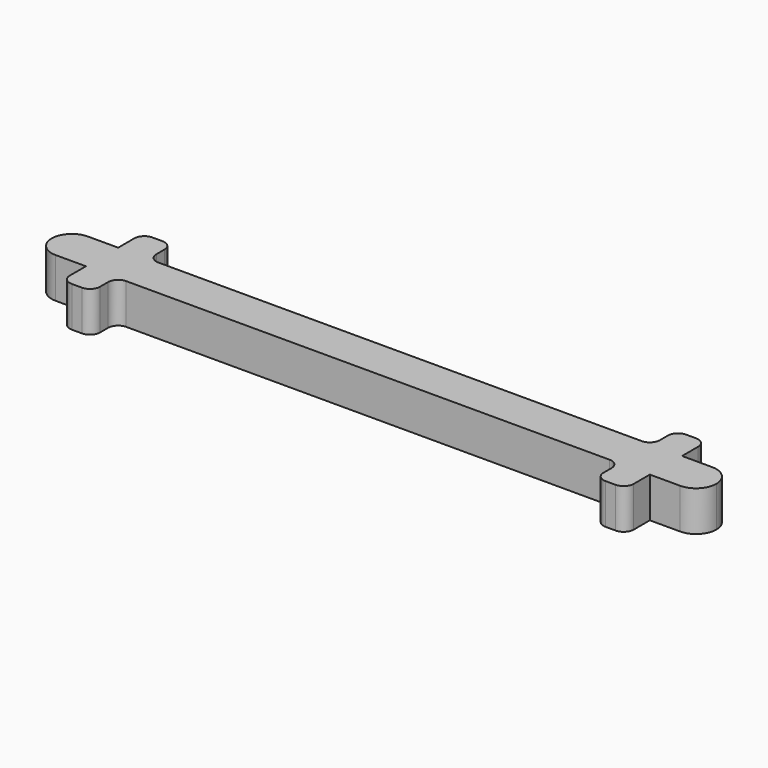
from build123d import *

# Parameters (mm, degrees)
F1_DEPTH = 4
F2_R     = 1.99999
F3_R     = 1


# Not quite as in the source:
# - a fillet or chamfer is up to 0.001 mm smaller than in the source, because OpenCascade refuses the exact size


with BuildPart() as f1:
    # F0 (on Top) → F1 (new body)
    with BuildSketch(Plane.XY):
        Polygon((-28, 2), (-33, 2), (-33, -2), (-28, -2), (-28, -5), (-25, -5), (-25, -2), (25, -2), (25, -5), (28, -5), (28, -2), (33, -2), (33, 2), (28, 2), (28, 5), (25, 5), (25, 2), (-25, 2), (-25, 5), (-28, 5), align=None)
    extrude(amount=F1_DEPTH)

    # F2 (radius 2 in the source; OpenCascade refuses exactly that, so slightly less here)
    f2_edges = [f1.edges().sort_by_distance(p)[0] for p in [
        (33, -2, 2),
        (33, 2, 2),
        (-33, -2, 2),
        (-33, 2, 2),
    ]]
    fillet(f2_edges, radius=F2_R)

    # F3
    f3_edges = [f1.edges().sort_by_distance(p)[0] for p in [
        (-28, -5, 2),
        (-28, 5, 2),
        (28, -5, 2),
        (28, 5, 2),
        (-25, -5, 2),
        (-25, 5, 2),
        (25, 5, 2),
        (25, -5, 2),
        (25, -2, 2),
        (25, 2, 2),
        (-25, 2, 2),
        (-25, -2, 2),
    ]]
    fillet(f3_edges, radius=F3_R)


solid = f1.part
